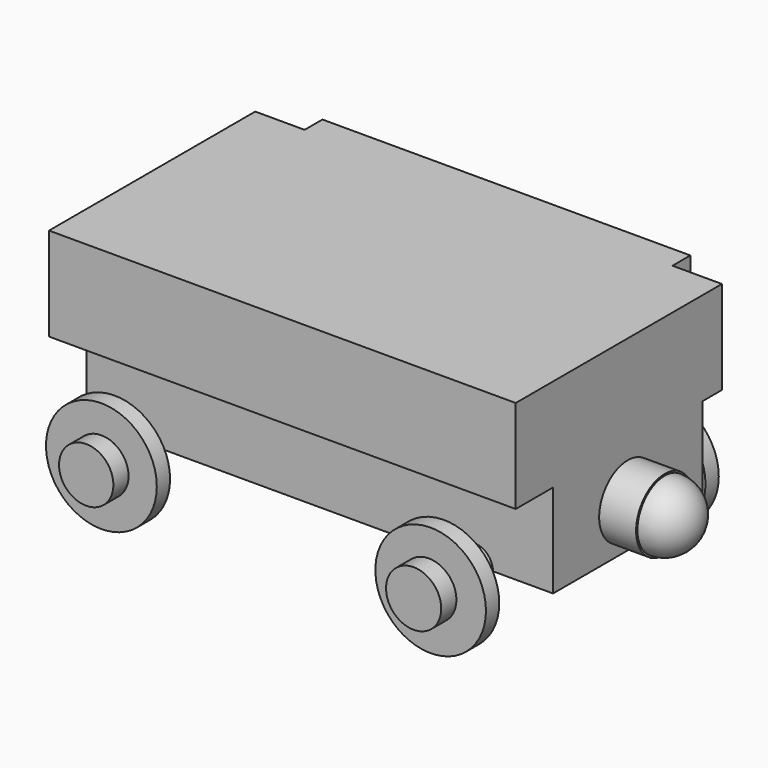
from build123d import *

# Parameters (mm, degrees)
F0_W      = 50
F0_H      = 20
F1_DEPTH  = 10
F2_W      = 50
F2_H      = 30
F3_DEPTH  = 10
F4_R      = 3.8263869055
F5_DEPTH  = 28.956
F10_W     = 5.2931006998
F10_H     = 2.3875854537
F10_W_2   = 5.2931062877
F11_DEPTH = 20.001
F12_R     = 1.7676057038
F12_R_2   = 2.0091255021
F13_DEPTH = 3.81
F14_R     = 5.9356630849
F14_R_2   = 5.9251919842
F15_DEPTH = 1.778
F16_R     = 2.9121930079
F16_R_2   = 2.9560346156
F17_DEPTH = 2.032


# Not quite as in the source:
# - a pattern or mirror of a feature is missing from the dataset's text; its kind, count and spacing are read off the source's solid


with BuildPart() as f1:
    # F0 (on Front) → F1 (new body, symmetric)
    with BuildSketch(Plane.XZ):
        Rectangle(F0_W, F0_H)
    extrude(amount=F1_DEPTH, both=True)

    # F2 (on Top) → F3 (join)
    with BuildSketch(Plane.XY):
        Rectangle(F2_W, F2_H)
    extrude(amount=F3_DEPTH)

    # F4 (on Right) → F5 (join, symmetric)
    with BuildSketch(Plane.YZ):
        with Locations((0, -5.3208619356)):
            Circle(F4_R)
    extrude(amount=F5_DEPTH, both=True)

    # F6 (on face) → F7 (revolve)
    with BuildSketch(Plane(origin=(-28.956, 0, 0), x_dir=(0, -1, 0), z_dir=(-1, 0, 0))):
        with BuildLine():
            Line((0, -1.5713692232), (0, -9.0703546481))
            ThreePointArc((0, -9.0703546481), (3.7494927125, -5.3208619356), (0, -1.5713692232))
        make_face()
    revolve(axis=Axis((-28.956, 0, -5.2824148391), (0, 0, -1)))

    # F8 (on face) → F9 (revolve)
    with BuildSketch(Plane.YZ.offset(28.956)):
        with BuildLine():
            Line((0, -1.6739376972), (0, -8.967786174))
            ThreePointArc((0, -8.967786174), (3.6469242384, -5.3208619356), (0, -1.6739376972))
        make_face()
    revolve(axis=Axis((28.956, 0, -5.3208619356), (0, 0, -1)))

    # F10 (on face) → F11 (cut, through all)
    with BuildSketch(Plane.XY.offset(10)):
        with Locations((-22.3534496501, 13.8062072732)):
            Rectangle(F10_W, F10_H)
        with Locations((22.3534468561, 13.8062072732)):
            Rectangle(F10_W_2, F10_H)
    extrude(amount=-F11_DEPTH, mode=Mode.SUBTRACT)

    # F12 (on face) → F13 (join)
    with BuildSketch(Plane.XZ.offset(10)):
        with Locations((-18.9186222851, -10)):
            Circle(F12_R)
        with Locations((16.5537931025, -10)):
            Circle(F12_R_2)
    f13 = extrude(amount=F13_DEPTH)

    # F13_copies: F13 across plane
    add(f13.mirror(Plane.ZX))

    # F14 (on face) → F15 (join)
    with BuildSketch(Plane.XZ.offset(13.81)):
        with Locations((-18.9186222851, -10)):
            Circle(F14_R)
        with Locations((16.3567233831, -10.247586295)):
            Circle(F14_R_2)
    f15 = extrude(amount=F15_DEPTH)

    # F15_copies: F15 across plane
    add(f15.mirror(Plane.ZX))

    # F16 (on face) → F17 (join)
    with BuildSketch(Plane.XZ.offset(15.588)):
        with Locations((-18.9186222851, -10)):
            Circle(F16_R)
        with Locations((16.1596573889, -10.247586295)):
            Circle(F16_R_2)
    f17 = extrude(amount=F17_DEPTH)

    # F17_copies: F17 across plane
    add(f17.mirror(Plane.ZX))


solid = f1.part
